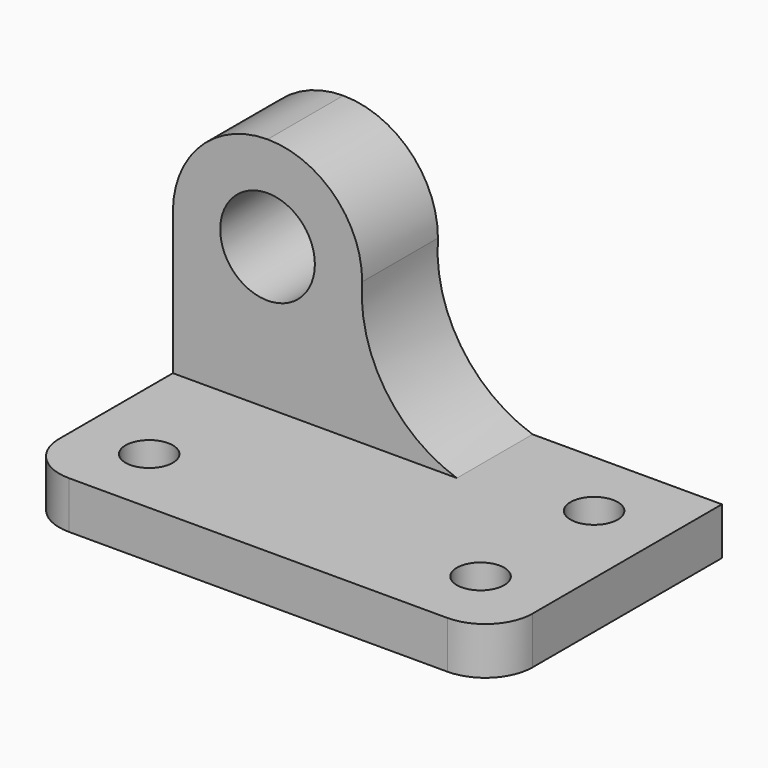
from build123d import *

# Parameters (mm, degrees)
F0_W      = 63.5
F0_H      = 38.1
F1_DEPTH  = 38.1
F3_DEPTH  = 31.75
F4_R      = 6.35
F5_DEPTH  = 44.45
F6_R      = 3.175
F7_DEPTH  = 25.4
F9_DEPTH  = 25.4
F11_DEPTH = 25.4


# Not quite as in the source:
# - a length typed as a fraction of an inch, garbled in the dataset ("3 / 203.2 mm" for 3/8 in), is restored


with BuildPart() as f1:
    # F0 (on Top) → F1 (new body)
    with BuildSketch(Plane.XY):
        with Locations((-10.9044740348, 19.05)):
            Rectangle(F0_W, F0_H)
    extrude(amount=F1_DEPTH)

    # F2 (on face) → F3 (cut)
    with BuildSketch(Plane.XY.offset(38.1)):
        Polygon((-4.5544740348, 25.4), (-42.6544740348, 25.4), (-42.6544740348, 0), (20.8455259652, 0), (20.8455259652, 38.1), (-4.5544740348, 38.1), align=None)
    extrude(amount=-F3_DEPTH, mode=Mode.SUBTRACT)

    # F4 (on face) → F5 (cut)
    with BuildSketch(Plane.XZ.offset(-25.4)):
        with Locations((-29.9544740348, 25.4)):
            Circle(F4_R)
        with BuildLine():
            ThreePointArc((-42.6544740348, 25.4), (-38.9347301559, 34.3802561211), (-29.9544740348, 38.1))
            Line((-29.9544740348, 38.1), (-42.6544740348, 38.1))
            Line((-42.6544740348, 38.1), (-42.6544740348, 25.4))
        make_face()
        with BuildLine():
            ThreePointArc((-29.9544740348, 38.1), (-20.9742179137, 34.3802561211), (-17.2544740348, 25.4))
            ThreePointArc((-17.2544740348, 25.4), (-14.2002037714, 13.6778468423), (-4.5544740348, 6.35))
            Line((-4.5544740348, 6.35), (-4.5544740348, 38.1))
            Line((-4.5544740348, 38.1), (-29.9544740348, 38.1))
        make_face()
    extrude(amount=-F5_DEPTH, mode=Mode.SUBTRACT)

    # F6 (on face) → F7 (cut)
    with BuildSketch(Plane.XY.offset(6.35)):
        with Locations((11.3205259652, 9.525)):
            Circle(F6_R)
        with Locations((-33.1294740348, 9.525)):
            Circle(F6_R)
        with Locations((11.3205259652, 28.575)):
            Circle(F6_R)
    extrude(amount=-F7_DEPTH, mode=Mode.SUBTRACT)

    # F8 (on face) → F9 (cut)
    with BuildSketch(Plane.XY.offset(6.35)):
        with BuildLine():
            ThreePointArc((-36.3044740348, 0), (-40.7946020953, 1.8598719395), (-42.6544740348, 6.35))
            Line((-42.6544740348, 6.35), (-42.6544740348, 0))
            Line((-42.6544740348, 0), (-36.3044740348, 0))
        make_face()
    extrude(amount=-F9_DEPTH, mode=Mode.SUBTRACT)

    # F10 (on face) → F11 (cut)
    with BuildSketch(Plane.XY.offset(6.35)):
        with BuildLine():
            Line((20.8455259652, 0), (20.8455259652, 6.35))
            ThreePointArc((20.8455259652, 6.35), (18.9856540257, 1.8598719395), (14.4955259652, 0))
            Line((14.4955259652, 0), (20.8455259652, 0))
        make_face()
    extrude(amount=-F11_DEPTH, mode=Mode.SUBTRACT)


solid = f1.part
